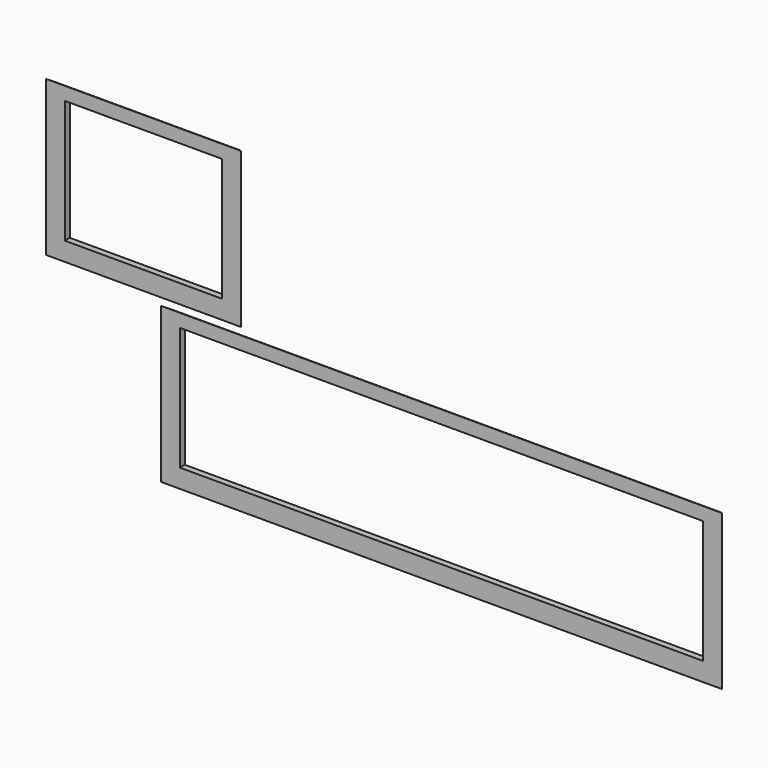
from build123d import *

# Parameters (mm, degrees)
F0_W     = 24
F0_H     = 12
F0_W_2   = 672
F0_H_2   = 158
F0_H_3   = 24
F1_DEPTH = 8
F3_DEPTH = 720
F4_SIZE  = 7.99999
F5_W     = 24
F5_H     = 24
F5_W_2   = 202
F5_H_2   = 158
F5_H_3   = 12
F6_DEPTH = 8
F8_DEPTH = 250
F9_SIZE  = 7.99999


# Not quite as in the source:
# - a fillet or chamfer is up to 0.001 mm smaller than in the source, because OpenCascade refuses the exact size


with BuildPart() as f1:
    # F0 (on Front) → F1 (new body)
    with BuildSketch(Plane.XZ):
        with Locations((-333.9108440578, 111.9455863265)):
            Rectangle(F0_W, F0_H)
        with Locations((14.0891559422, 111.9455863265)):
            Rectangle(F0_W_2, F0_H)
        with Locations((-333.9108440578, 26.9455863265)):
            Rectangle(F0_W, F0_H_2)
        with Locations((-333.9108440578, -64.0544136735)):
            Rectangle(F0_W, F0_H_3)
        with Locations((14.0891559422, -64.0544136735)):
            Rectangle(F0_W_2, F0_H_3)
        with Locations((362.0891559422, 111.9455863265)):
            Rectangle(F0_W, F0_H)
        with Locations((362.0891559422, 26.9455863265)):
            Rectangle(F0_W, F0_H_2)
        with Locations((362.0891559422, -64.0544136735)):
            Rectangle(F0_W, F0_H_3)
    extrude(amount=F1_DEPTH)

    # F2 (on face) → F3 (join)
    with BuildSketch(Plane.YZ.offset(374.0891559422)):
        Polygon((-8, 122.9455863265), (-8, 117.9455863265), (0, 117.9455863265), align=None)
    extrude(amount=-F3_DEPTH)

    # F4 (size 8 in the source; OpenCascade refuses exactly that, so slightly less here)
    f4_edges = [f1.edges().sort_by_distance(p)[0] for p in [
        (374.089156, 0, 20.945586),
        (-345.910844, 0, 20.945586),
    ]]
    chamfer(f4_edges, length=F4_SIZE)


with BuildPart() as f6:
    # F5 (on Front) → F6 (new body)
    with BuildSketch(Plane.XZ):
        with Locations((-255.5729791075, 144.4389531016)):
            Rectangle(F5_W, F5_H)
        with Locations((-368.5729791075, 144.4389531016)):
            Rectangle(F5_W_2, F5_H)
        with Locations((-255.5729791075, 235.4389531016)):
            Rectangle(F5_W, F5_H_2)
        with Locations((-481.5729791075, 144.4389531016)):
            Rectangle(F5_W, F5_H)
        with Locations((-255.5729791075, 320.4389531016)):
            Rectangle(F5_W, F5_H_3)
        with Locations((-481.5729791075, 235.4389531016)):
            Rectangle(F5_W, F5_H_2)
        with Locations((-368.5729791075, 320.4389531016)):
            Rectangle(F5_W_2, F5_H_3)
        with Locations((-481.5729791075, 320.4389531016)):
            Rectangle(F5_W, F5_H_3)
    extrude(amount=F6_DEPTH)

    # F7 (on face) → F8 (join)
    with BuildSketch(Plane(origin=(-493.5729791075, 0, 0), x_dir=(0, -1, 0), z_dir=(-1, 0, 0))):
        Polygon((0, 326.4389531016), (8, 326.4389531016), (8, 331.4389531016), align=None)
    extrude(amount=-F8_DEPTH)

    # F9 (size 8 in the source; OpenCascade refuses exactly that, so slightly less here)
    f9_edges = [f6.edges().sort_by_distance(p)[0] for p in [
        (-493.572979, 0, 229.438953),
        (-243.572979, 0, 229.438953),
    ]]
    chamfer(f9_edges, length=F9_SIZE)


solid = Compound([f1.part, f6.part])
